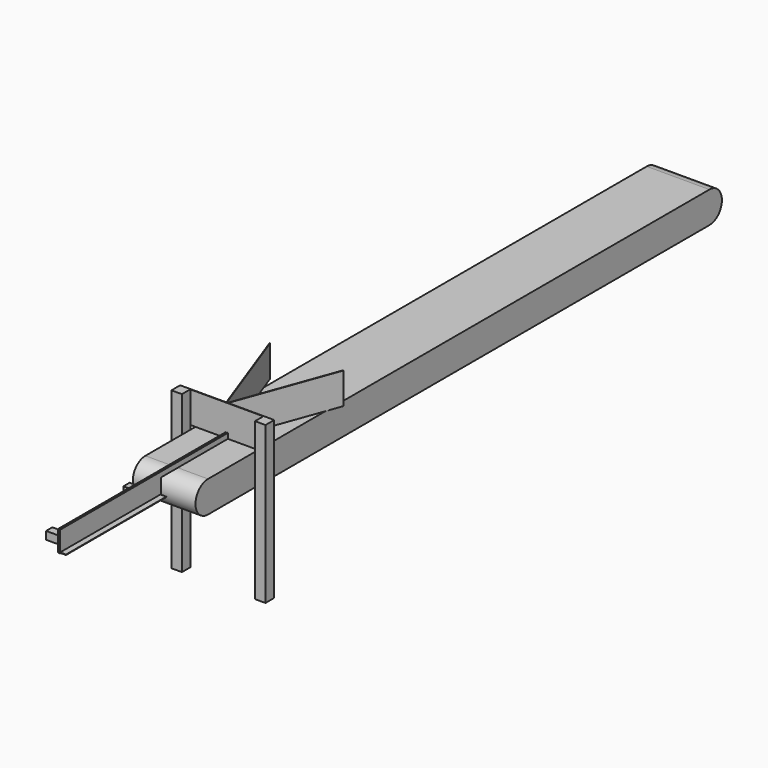
from build123d import *

# Parameters (mm, degrees)
F1_DEPTH      = 304.8
F3_DEPTH      = 152.4
F2_W          = 50.8
F2_H          = 50.8
F4_DEPTH      = 152.4
F4_DEPTH_BACK = 609.6
F8_W          = 4.064
F8_H          = 2.54
F9_DEPTH      = 2.286
F10_W         = 3.175
F10_H         = 304.8
F10_H_2       = 101.6
F11_DEPTH     = 25.4
F12_W         = 3.175
F12_H         = 609.6
F13_DEPTH     = 101.6
F12_W_2       = 4.064
F12_W_3       = 25.4
F14_DEPTH     = 2.286
F15_W         = 38.1
F15_H         = 38.1
F16_DEPTH     = 101.6
F18_DEPTH     = 3.175


# Not quite as in the source:
# - a feature of the source that left no trace in its solid (it failed there, or was rolled back) is left out
# - a pattern or mirror of a feature is missing from the dataset's text; its kind, count and spacing are read off the source's solid


with BuildPart() as f1:
    # F0 (on Right) → F1 (new body)
    with BuildSketch(Plane.YZ):
        with BuildLine():
            Line((1567.5077411821, 76.3827925089), (-1480.4922588179, 76.3827925089))
            ThreePointArc((-1480.4922588179, 76.3827925089), (-1556.6922588179, 0.1827925089), (-1480.4922588179, -76.0172074911))
            Line((-1480.4922588179, -76.0172074911), (1567.5077411821, -76.0172074911))
            ThreePointArc((1567.5077411821, -76.0172074911), (1643.7077411821, 0.1827925089), (1567.5077411821, 76.3827925089))
        make_face()
    extrude(amount=F1_DEPTH)

    # F2 (on face) → F3 (join)
    with BuildSketch(Plane.XY.offset(76.3827925089)):
        Polygon((330.2, -1175.6922588179), (381, -1175.6922588179), (381, -1173.4062588179), (304.8, -1173.4062588179), (304.8, -1175.6922588179), align=None)
        Polygon((152.4, -1175.6922588179), (304.8, -1175.6922588179), (304.8, -1173.4062588179), (156.8647103879, -1173.4062588179), (154.432, -1173.4062588179), (152.4, -1173.4062588179), align=None)
        Polygon((304.8, -760.2735742093), (304.8, -766.9573910681), (332.3481373311, -691.2695058028), (330.2, -690.4876477552), align=None)
        Polygon((154.432, -1173.4062588179), (156.8647103879, -1173.4062588179), (304.8, -766.9573910681), (304.8, -760.2735742093), align=None)
    f3 = extrude(amount=F3_DEPTH)

    # F3_copies: F3 across plane
    add(f3.mirror(Plane(origin=(152.4, 0, 0), x_dir=(0, 0, -1), z_dir=(-1, 0, 0))))

    # F2 (on face) → F4 (join, two sides)
    with BuildSketch(Plane.XY.offset(76.3827925089)) as f4_sk:
        with Locations((355.6, -1201.0922588179)):
            Rectangle(F2_W, F2_H)
    f4 = extrude(amount=F4_DEPTH) + extrude(f4_sk.sketch, amount=-F4_DEPTH_BACK)

    # F4_copies: F4 across plane
    add(f4.mirror(Plane(origin=(152.4, 0, 0), x_dir=(0, 0, -1), z_dir=(-1, 0, 0))))

    # F8 (on face) → F9 (cut, through all)
    with BuildSketch(Plane(origin=(0, -1173.4062588179, 0), x_dir=(-1, 0, 0), z_dir=(0, 1, 0))):
        with Locations((-152.4, 77.6527925089)):
            Rectangle(F8_W, F8_H)
    extrude(amount=-F9_DEPTH, mode=Mode.SUBTRACT)

    # F10 (on face) → F11 (join)
    with BuildSketch(Plane.XY.offset(76.3827925089)):
        with Locations((156.0195, -1328.0922588179)):
            Rectangle(F10_W, F10_H)
        with Locations((148.7805, -1328.0922588179)):
            Rectangle(F10_W, F10_H)
        with Locations((156.0195, -1531.2922588179)):
            Rectangle(F10_W, F10_H_2)
        with Locations((148.7805, -1531.2922588179)):
            Rectangle(F10_W, F10_H_2)
    extrude(amount=F11_DEPTH)

    # F12 (on Top) → F13 (join)
    with BuildSketch(Plane.XY):
        with Locations((148.7805, -1886.8922588179)):
            Rectangle(F12_W, F12_H)
        with Locations((156.0195, -1886.8922588179)):
            Rectangle(F12_W, F12_H)
        Polygon((154.432, -2191.6922588179), (150.368, -2191.6922588179), (147.193, -2191.6922588179), (147.193, -2194.8672588179), (157.607, -2194.8672588179), (157.607, -2191.6922588179), align=None)
    extrude(amount=F13_DEPTH)

    # F12 (on Top) → F14 (join)
    with BuildSketch(Plane.XY):
        with Locations((152.4, -1886.8922588179)):
            Rectangle(F12_W_2, F12_H)
        with Locations((170.307, -1886.8922588179)):
            Rectangle(F12_W_3, F12_H)
        with Locations((156.0195, -1886.8922588179)):
            Rectangle(F12_W, F12_H)
    extrude(amount=F14_DEPTH)

    # F15 (on face) → F16 (join)
    with BuildSketch(Plane(origin=(147.193, 0, 0), x_dir=(0, -1, 0), z_dir=(-1, 0, 0))):
        with Locations((1651.9422588179, 19.05)):
            Rectangle(F15_W, F15_H)
        with Locations((2121.8422588179, 19.05)):
            Rectangle(F15_W, F15_H)
    extrude(amount=F16_DEPTH)

    # F17 (on face) → F18 (cut, through all)
    with BuildSketch(Plane.YZ.offset(157.607)):
        Polygon((-2192.5812588179, 4.826), (-2192.5812588179, 2.286), (-2191.6922588179, 2.286), (-1582.0922588179, 2.286), (-1582.0922588179, 4.826), align=None)
    extrude(amount=-F18_DEPTH, mode=Mode.SUBTRACT)


solid = f1.part
